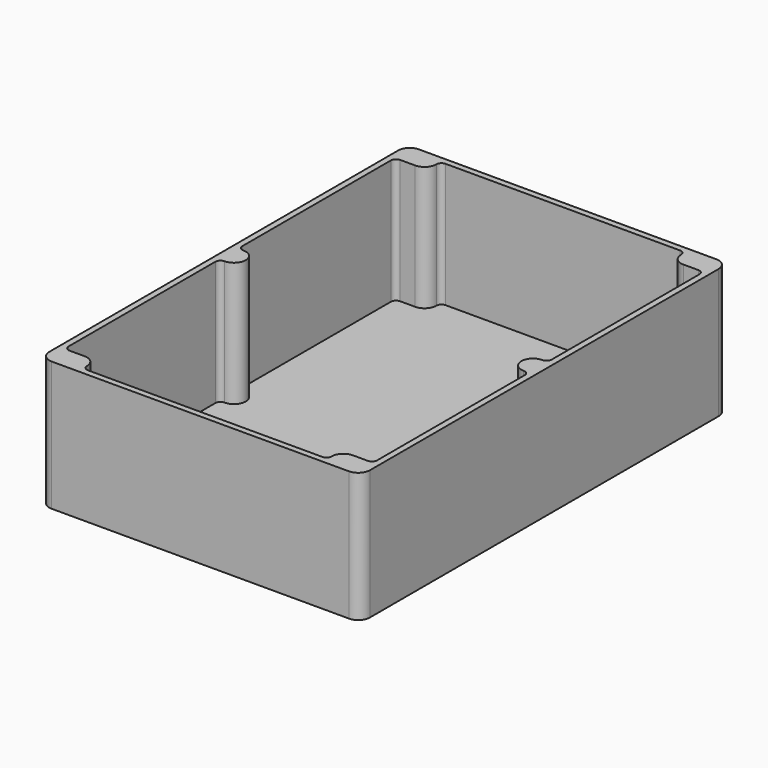
from build123d import *

# Parameters (mm, degrees)
F1_DEPTH = 3
F0_W     = 185
F0_H     = 265
F2_DEPTH = 74.8
F3_R     = 6.75
F4_R     = 2.99999


# Not quite as in the source:
# - a fillet or chamfer is up to 0.001 mm smaller than in the source, because OpenCascade refuses the exact size
# - ends of sketch curves that miss each other by under 0.0002 mm in the source are joined


with BuildPart() as f1:
    # F0 (on Top) → F1 (new body)
    with BuildSketch(Plane.XY):
        with BuildLine():
            Line((70.6, 125.95), (70.6, 129))
            Line((70.6, 129), (-70.6, 129))
            Line((-70.6, 129), (-70.6, 125.95))
            ThreePointArc((-70.6, 125.95), (-72.577029227, 121.177029227), (-77.35, 119.2))
            Line((-77.35, 119.2), (-89, 119.2))
            Line((-89, 119.2), (-89, 6.080118008))
            Line((-89, 6.080118008), (-86, 6.080118008))
            ThreePointArc((-86, 6.080118008), (-79.25, -0.669881992), (-86, -7.419881992))
            Line((-86, -7.419881992), (-89, -7.419881992))
            Line((-89, -7.419881992), (-89, -119.2))
            Line((-89, -119.2), (-77.3450501441, -119.2))
            ThreePointArc((-77.3450501441, -119.2), (-72.4815603684, -121.2692984284), (-70.6, -126.2084541623))
            Line((-70.6, -126.2084541623), (-70.6, -129))
            Line((-70.6, -129), (70.6, -129))
            Line((70.6, -129), (70.6, -125.95))
            ThreePointArc((70.6, -125.95), (72.577029227, -121.177029227), (77.35, -119.2))
            Line((77.35, -119.2), (89, -119.2))
            Line((89, -119.2), (89, -6.75))
            Line((89, -6.75), (86, -6.75))
            ThreePointArc((86, -6.75), (79.25, 0), (86, 6.75))
            Line((86, 6.75), (89, 6.75))
            Line((89, 6.75), (89, 119.2))
            Line((89, 119.2), (77.35, 119.2))
            ThreePointArc((77.35, 119.2), (72.577029227, 121.177029227), (70.6, 125.95))
        make_face()
    extrude(amount=F1_DEPTH)

    # F0 (on Top) → F2 (join)
    with BuildSketch(Plane.XY):
        Rectangle(F0_W, F0_H)
        Polygon((70.6, 129), (89, 129), (89, 119.2), (89, 6.75), (89, -6.75), (89, -119.2), (89, -129), (70.6, -129), (-70.6, -129), (-89, -129), (-89, -119.2), (-89, -7.419881992), (-89, 6.080118008), (-89, 119.2), (-89, 129), (-70.6, 129), align=None, mode=Mode.SUBTRACT)
        with BuildLine():
            Line((-77.3450501441, -119.2), (-89, -119.2))
            Line((-89, -119.2), (-89, -129))
            Line((-89, -129), (-70.6, -129))
            Line((-70.6, -129), (-70.6, -126.2084541623))
            ThreePointArc((-70.6, -126.2084541623), (-72.4815603684, -121.2692984284), (-77.3450501441, -119.2))
        make_face()
        with BuildLine():
            Line((89, -129), (89, -119.2))
            Line((89, -119.2), (77.35, -119.2))
            ThreePointArc((77.35, -119.2), (72.577029227, -121.177029227), (70.6, -125.95))
            Line((70.6, -125.95), (70.6, -129.000006485))
            Line((70.6, -129.000006485), (89, -129))
        make_face()
        with BuildLine():
            Line((-70.6, 125.95), (-70.6, 129))
            Line((-70.6, 129), (-89, 129))
            Line((-89, 129), (-89, 119.2))
            Line((-89, 119.2), (-77.35, 119.2))
            ThreePointArc((-77.35, 119.2), (-72.577029227, 121.177029227), (-70.6, 125.95))
        make_face()
        with BuildLine():
            Line((89, 119.2), (89, 129))
            Line((89, 129), (70.6, 129))
            Line((70.6, 129), (70.6, 125.95))
            ThreePointArc((70.6, 125.95), (72.577029227, 121.177029227), (77.35, 119.2))
            Line((77.35, 119.2), (89, 119.2))
        make_face()
        with BuildLine():
            Line((-86, 6.080118008), (-89, 6.080118008))
            Line((-89, 6.080118008), (-89, -7.419881992))
            Line((-89, -7.419881992), (-86, -7.419881992))
            ThreePointArc((-86, -7.419881992), (-79.25, -0.669881992), (-86, 6.080118008))
        make_face()
        with BuildLine():
            Line((89, -6.75), (89, 6.75))
            Line((89, 6.75), (86, 6.75))
            ThreePointArc((86, 6.75), (79.25, 0), (86, -6.75))
            Line((86, -6.75), (89, -6.75))
        make_face()
    extrude(amount=F2_DEPTH)

    # F3
    f3_edges = [f1.edges().sort_by_distance(p)[0] for p in [
        (-92.5, 132.5, 37.4),
        (92.5, 132.5, 37.4),
        (92.5, -132.5, 37.4),
        (-92.5, -132.5, 37.4),
    ]]
    fillet(f3_edges, radius=F3_R)

    # F4 (radius 3 in the source; OpenCascade refuses exactly that, so slightly less here)
    f4_edges = [f1.edges().sort_by_distance(p)[0] for p in [
        (-89, 6.080118, 38.9),
        (-89, 119.2, 38.9),
        (-70.6, 129, 38.9),
        (70.6, 129, 38.9),
        (89, 119.2, 38.9),
        (-89, -7.419882, 38.9),
        (89, 6.75, 38.9),
        (89, -6.75, 38.9),
        (-89, -119.2, 38.9),
        (-70.6, -129, 38.9),
        (70.6, -129, 38.9),
        (89, -119.2, 38.9),
    ]]
    fillet(f4_edges, radius=F4_R)


solid = f1.part
